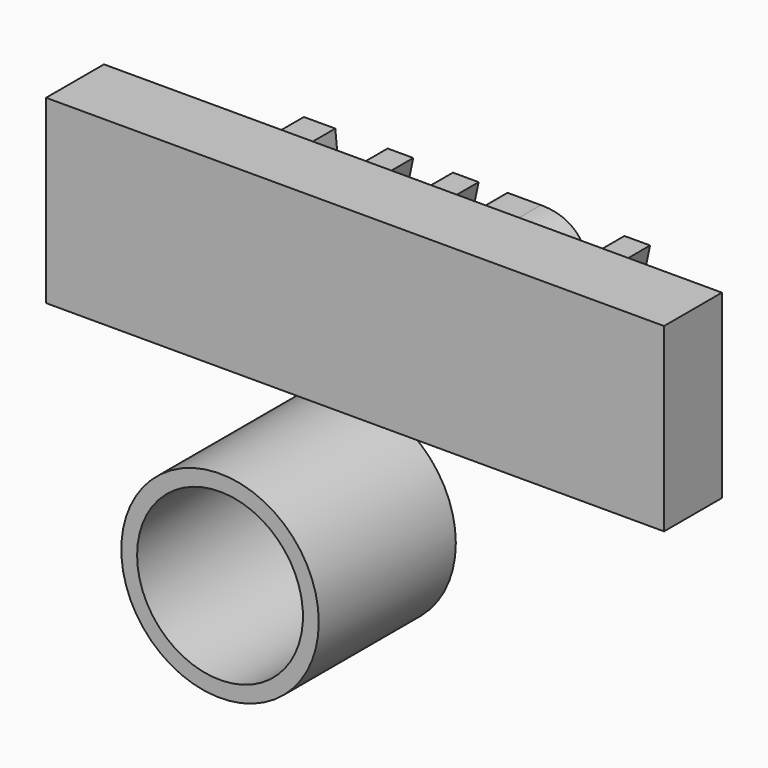
from build123d import *

# Parameters (mm, degrees)
F0_TEXT_SIZE = 22.9948096805
F1_DEPTH     = 16.764
F2_W         = 82.4530534446
F2_H         = 24.1251531988
F3_DEPTH     = 9.652
F4_R         = 13.1739527637
F5_DEPTH     = 22.86
F6_R         = 11.3362004223
F7_DEPTH     = 64.516
F8_R         = 12.0190084583
F9_DEPTH     = 40.894
F10_R        = 10.6665212218
F11_DEPTH    = 33.02
F12_R        = 11.0656086281
F13_DEPTH    = 84.582


# Not quite as in the source:
# - Text() gives the source's letters only with a copy of the font that has no kerning and outlines rounded to 1/6400 em; it was checked with that copy


with BuildPart() as f1:
    # F0 (on Front) → F1 (new body)
    with BuildSketch(Plane.XZ):
        with Locations((-47.7664843202, 22.3417282104)):
            Text('AUDI', F0_TEXT_SIZE, font='Open Sans', font_style=FontStyle.BOLDITALIC, text_align=(TextAlign.LEFT, TextAlign.BOTTOM))
    extrude(amount=-F1_DEPTH)

    # F6 (on face) → F7 (cut)
    with BuildSketch(Plane.XZ):
        with Locations((-38.3253991604, -8.7033780292)):
            Circle(F6_R)
    extrude(amount=F7_DEPTH, mode=Mode.SUBTRACT)

    # F8 (on face) → F9 (cut)
    with BuildSketch(Plane.XZ):
        with Locations((-38.3253991604, -8.7033780292)):
            Circle(F8_R)
    extrude(amount=F9_DEPTH, mode=Mode.SUBTRACT)

    # F10 (on face) → F11 (cut)
    with BuildSketch(Plane.XZ):
        with Locations((-38.3253991604, -8.7033780292)):
            Circle(F10_R)
    extrude(amount=F11_DEPTH, mode=Mode.SUBTRACT)


with BuildPart() as f3:
    # F2 (on Front) → F3 (new body)
    with BuildSketch(Plane.XZ):
        with Locations((-20.3078817576, 29.0112597868)):
            Rectangle(F2_W, F2_H)
    extrude(amount=-F3_DEPTH)


with BuildPart() as f5:
    # F4 (on Front) → F5 (new body)
    with BuildSketch(Plane.XZ):
        with Locations((-38.3253991604, -8.7033780292)):
            Circle(F4_R)
    extrude(amount=-F5_DEPTH)

    # F12 (on face) → F13 (cut)
    with BuildSketch(Plane(origin=(0, 22.86, 0), x_dir=(-1, 0, 0), z_dir=(0, 1, 0))):
        with Locations((38.3253991604, -8.7033780292)):
            Circle(F12_R)
    extrude(amount=-F13_DEPTH, mode=Mode.SUBTRACT)


solid = Compound([f1.part, f3.part, f5.part])
